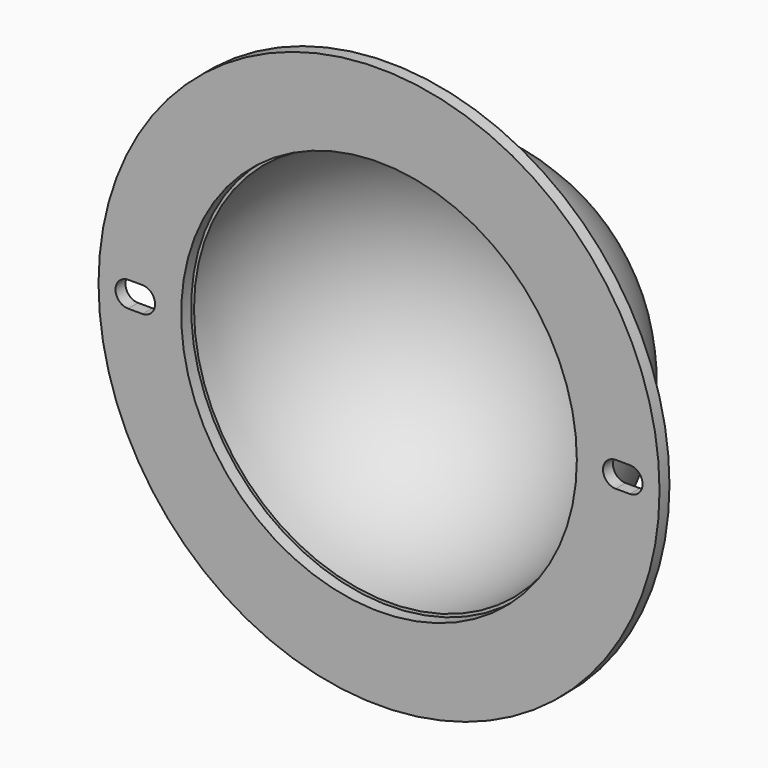
from build123d import *

# Parameters (mm, degrees)
F0_R     = 49.625
F0_R_2   = 35
F1_DEPTH = 2.2
F4_T     = 2.5


# Not quite as in the source:
# - a shell that OpenCascade refuses in one call is made with other operations: the cavity is built on its own and cut out
# - a feature names something its author has since deleted; it is built from what else it names


with BuildPart() as f1:
    # F0 (on Front) → F1 (new body)
    with BuildSketch(Plane.XZ):
        Circle(F0_R)
        with BuildLine():
            ThreePointArc((-44.375, -2.25), (-46.625, 0), (-44.375, 2.25))
            Line((-44.375, 2.25), (-41.875, 2.25))
            ThreePointArc((-41.875, 2.25), (-39.625, 0), (-41.875, -2.25))
            Line((-41.875, -2.25), (-44.375, -2.25))
        make_face(mode=Mode.SUBTRACT)
        Circle(F0_R_2, mode=Mode.SUBTRACT)
        with BuildLine():
            Line((44.375, -2.25), (41.875, -2.25))
            ThreePointArc((41.875, -2.25), (39.625, 0), (41.875, 2.25))
            Line((41.875, 2.25), (44.375, 2.25))
            ThreePointArc((44.375, 2.25), (46.625, 0), (44.375, -2.25))
        make_face(mode=Mode.SUBTRACT)
    extrude(amount=F1_DEPTH)

    # F2 (on Top) → F3 (revolve)
    with BuildSketch(Plane.XY):
        with BuildLine():
            Line((0, 0), (37, 0))
            ThreePointArc((37, 0), (26.1629509039, 26.1629509039), (0, 37))
            Line((0, 37), (0, 0))
        make_face()
    revolve(axis=Axis((0, 18.5, 0), (0, 1, 0)))

    # F4: shell of thickness 2.5, made by hand


with BuildPart() as f4_core1:
    # F4_t2: copy of F1
    add(f1.part)

    # the walls: a layer under each face that stays
    f4_faces = [f4_core1.faces().sort_by_distance(p)[0] for p in [
        (-49.625, -1.1, 0),
        (-33.0833333333, 0, -33.0833333333),
        (-33.0833333333, -2.2, -33.0833333333),
        (-46.625, -1.1, 0),
        (-43.125, -1.1, -2.25),
        (-43.125, -1.1, 2.25),
        (-39.625, -1.1, 0),
        (-26.1629509039, 26.1629509039, 0),
        (43.125, -1.1, -2.25),
        (46.625, -1.1, 0),
        (39.625, -1.1, 0),
        (43.125, -1.1, 2.25),
        (-35, -1.1, 0),
    ]]
    thicken(f4_faces, amount=-F4_T, mode=Mode.SUBTRACT)

    # F4_s3 → F4_t4 (revolve, cut)
    with BuildSketch(Plane.XY):
        Polygon((37.025, 0.025), (37, -2.5), (34.5, -2.5), (34.5, 0), align=None)
    revolve(axis=Axis((0, 0, 0), (0, 1, 0)), mode=Mode.SUBTRACT)


with BuildPart() as f1_1:
    add(f1.part)

    # what is left inside the walls is the cavity
    f4_cavity = [f4_core1.part.solids().sort_by_distance(p)[0] for p in [
        (-29.856226, 17.2375, 0),
    ]]
    add(f4_cavity, mode=Mode.SUBTRACT)


solid = f1_1.part
